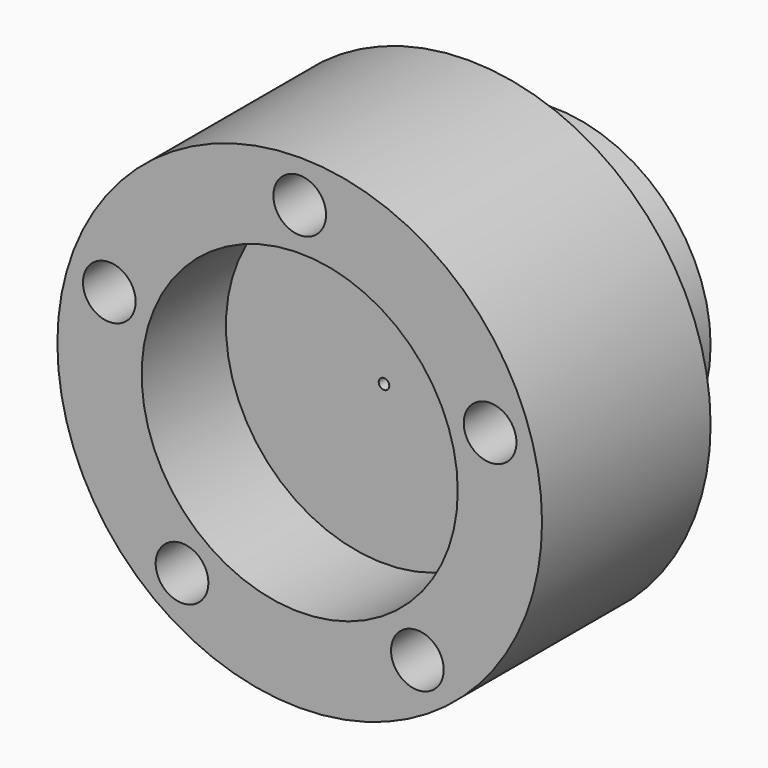
from build123d import *

# Parameters (mm, degrees)
F0_R     = 115
F0_R_2   = 12.5
F0_R_3   = 75
F1_DEPTH = 100
F2_DEPTH = 50
F3_DEPTH = 50
F4_R     = 12.5
F5_DEPTH = 25
F6_DEPTH = 99
F7_R     = 2.5
F8_DEPTH = 150.001


with BuildPart() as f1:
    # F0 (on Front) → F1 (new body)
    with BuildSketch(Plane.XZ):
        Circle(F0_R)
        with Locations((-55.8395989678, -76.8566144656)):
            Circle(F0_R_2, mode=Mode.SUBTRACT)
        with Locations((55.8395989678, -76.8566144656)):
            Circle(F0_R_2, mode=Mode.SUBTRACT)
        with Locations((-90.350369048, 29.3566144656)):
            Circle(F0_R_2, mode=Mode.SUBTRACT)
        Circle(F0_R_3, mode=Mode.SUBTRACT)
        with Locations((90.350369048, 29.3566144656)):
            Circle(F0_R_2, mode=Mode.SUBTRACT)
        with Locations((0, 95)):
            Circle(F0_R_2, mode=Mode.SUBTRACT)
    extrude(amount=F1_DEPTH)

    # F4 (on face) → F5 (cut)
    with BuildSketch(Plane(origin=(0, 50, 0), x_dir=(-1, 0, 0), z_dir=(0, 1, 0))):
        Circle(F4_R)
    extrude(amount=F5_DEPTH, mode=Mode.SUBTRACT)


with BuildPart() as f2:
    # F0 (on Front) → F2 (new body)
    with BuildSketch(Plane.XZ):
        Circle(F0_R_3)
    extrude(amount=-F2_DEPTH)

    # F4 (on face) → F6 (cut)
    with BuildSketch(Plane(origin=(0, 50, 0), x_dir=(-1, 0, 0), z_dir=(0, 1, 0))):
        Circle(F4_R)
    extrude(amount=-F6_DEPTH, mode=Mode.SUBTRACT)


with BuildPart() as f3:
    # F0 (on Front) → F3 (new body)
    with BuildSketch(Plane.XZ):
        Circle(F0_R_3)
    extrude(amount=F3_DEPTH)

    # F7 (on face) → F8 (cut, through all)
    with BuildSketch(Plane(origin=(0, 50, 0), x_dir=(-1, 0, 0), z_dir=(0, 1, 0))):
        Circle(F7_R)
    extrude(amount=-F8_DEPTH, mode=Mode.SUBTRACT)


solid = Compound([f1.part, f2.part, f3.part])
